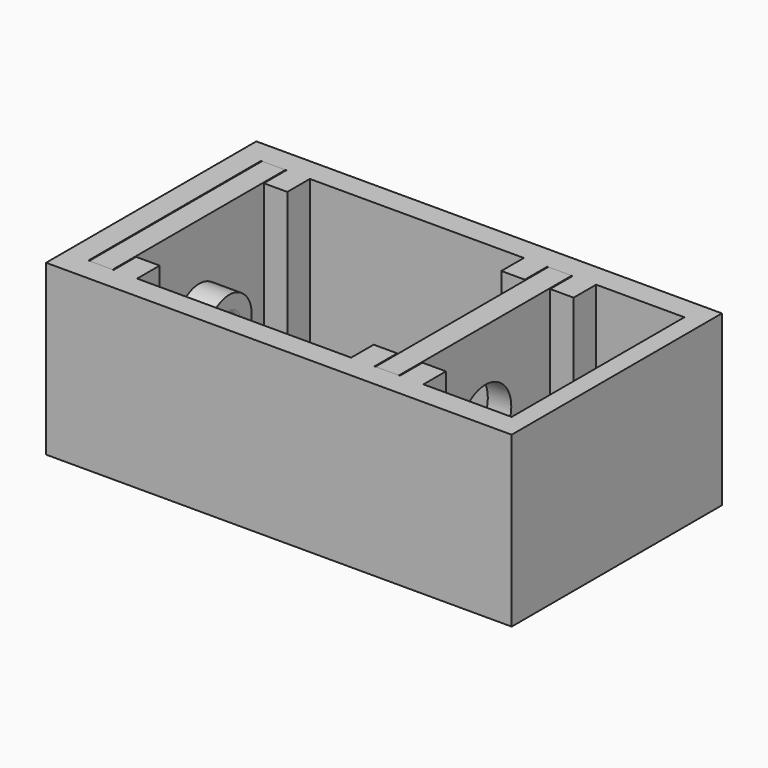
from build123d import *

# Parameters (mm, degrees)
F0_W      = 33
F0_H      = 23
F0_W_2    = 28
F0_H_2    = 18
F1_DEPTH  = 18
F2_R      = 3.45
F3_DEPTH  = 5
F4_R      = 3
F5_DEPTH  = 3.2
F6_R      = 1
F7_DEPTH  = 1
F8_R      = 0.49999
F9_W      = 2.5
F9_H      = 3
F10_DEPTH = 18
F11_W     = 28
F11_H     = 2.5
F12_DEPTH = 25


# Not quite as in the source:
# - a fillet or chamfer is up to 0.001 mm smaller than in the source, because OpenCascade refuses the exact size


with BuildPart() as f1:
    # F0 (on Top) → F1 (new body)
    with BuildSketch(Plane.XY):
        Rectangle(F0_W, F0_H)
        Rectangle(F0_W_2, F0_H_2, mode=Mode.SUBTRACT)
    extrude(amount=F1_DEPTH)

    # F2 (on face) → F3 (cut)
    with BuildSketch(Plane.YZ.offset(16.5)):
        with Locations((0, 9)):
            Circle(F2_R)
    extrude(amount=-F3_DEPTH, mode=Mode.SUBTRACT)

    # F4 (on face) → F5 (join)
    with BuildSketch(Plane.YZ.offset(-14)):
        with Locations((0, 9)):
            Circle(F4_R)
    extrude(amount=F5_DEPTH)

    # F6 (on face) → F7 (cut)
    with BuildSketch(Plane.YZ.offset(-10.8)):
        with Locations((0, 9)):
            Circle(F6_R)
    extrude(amount=-F7_DEPTH, mode=Mode.SUBTRACT)

    # F8 (radius 0.5 in the source; OpenCascade refuses exactly that, so slightly less here)
    f8_edges = [f1.edges().sort_by_distance(p)[0] for p in [
        (-11.8, -1, 9),
        (-10.8, -1, 9),
    ]]
    fillet(f8_edges, radius=F8_R)

    # F11 (on face) → F12 (cut)
    with BuildSketch(Plane(origin=(0, 0, 0), x_dir=(1, 0, 0), z_dir=(0, 0, -1))):
        with Locations((0, -10.25)):
            Rectangle(F11_W, F11_H)
        with Locations((0, 10.25)):
            Rectangle(F11_W, F11_H)
        Polygon((-14, -9), (14, -9), (14, 9), (-14, 9), (-14, 4.632844124), (-9.7779119387, 4.632844124), (-9.7779119387, -4.2528109625), (-14, -4.2528109625), align=None)
    extrude(amount=-F12_DEPTH, mode=Mode.SUBTRACT)


with BuildPart() as f10:
    # F9 (on Top) → F10 (new body)
    with BuildSketch(Plane.XY):
        Polygon((-19.1, 0), (-16.6, 0), (-16.6, 11.5), (-13.9, 11.5), (-13.9, 8.5), (-11.4, 8.5), (-11.4, 11.5), (11.4, 11.5), (11.4, 8.5), (13.9, 8.5), (13.9, 11.5), (16.6, 11.5), (19.1, 11.5), (28.5, 11.5), (28.5, 0), (30.5, 0), (30.5, 14), (-19.1, 14), align=None)
        Polygon((-16.6, -11.5), (-16.6, 0), (-19.1, 0), (-19.1, -14), (30.5, -14), (30.5, 0), (28.5, 0), (28.5, -11.5), (19.1, -11.5), (16.6, -11.5), (13.9, -11.5), (13.9, -8.5), (11.4, -8.5), (11.4, -11.5), (-11.4, -11.5), (-11.4, -8.5), (-13.9, -8.5), (-13.9, -11.5), align=None)
        with Locations((17.85, 10)):
            Rectangle(F9_W, F9_H)
        with Locations((17.85, -10)):
            Rectangle(F9_W, F9_H)
    extrude(amount=F10_DEPTH)


solid = Compound([f1.part, f10.part])
